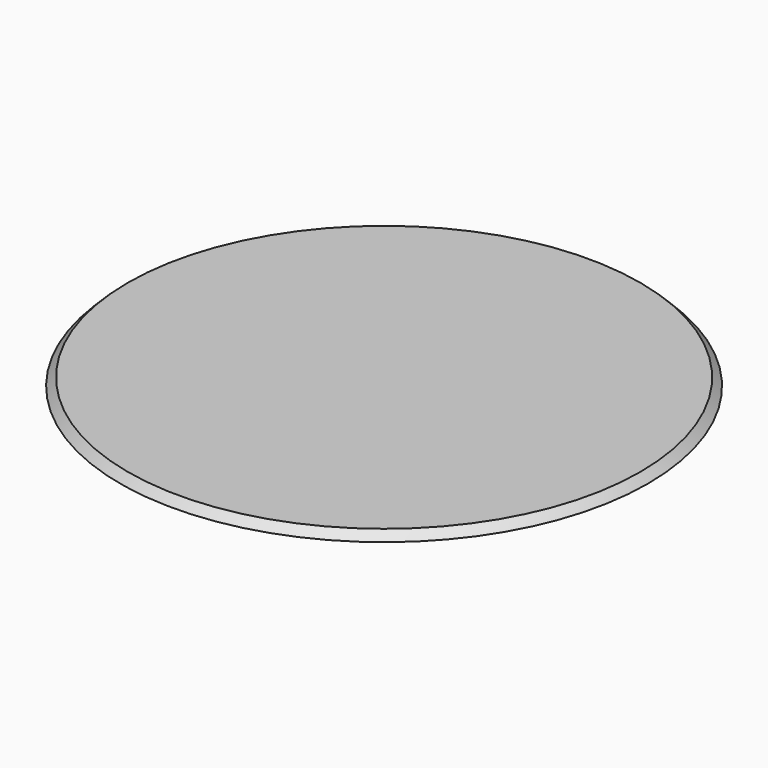
from build123d import *

# Parameters (mm, degrees)
F0_R     = 571.5
F1_DEPTH = 12.7
F2_DEPTH = 3.81


# Not quite as in the source:
# - a fillet or chamfer that OpenCascade refuses, or shapes differently, is made with other operations: its cross-section is extruded or revolved along the edge and cut away or added


with BuildPart() as f1:
    # F0 (on Top) → F1 (new body)
    with BuildSketch(Plane.XY):
        Circle(F0_R)
    extrude(amount=F1_DEPTH)

    # F2 (add): a face of the model
    f2_faces = [f1.faces().sort_by_distance(p)[0] for p in [
        (0, 0, 12.7),
    ]]
    extrude(f2_faces, amount=F2_DEPTH)

    # F3: chamfer of 25.4 on 1 edges, made by hand

    # F3_s1 → F3_t2 (revolve, cut)
    with BuildSketch(Plane.XZ):
        Polygon((571.5, -8.89), (546.1, 16.51), (571.5, 16.51), align=None)
    revolve(axis=Axis((0, 0, 16.51), (0, 0, 1)), mode=Mode.SUBTRACT)


solid = f1.part
